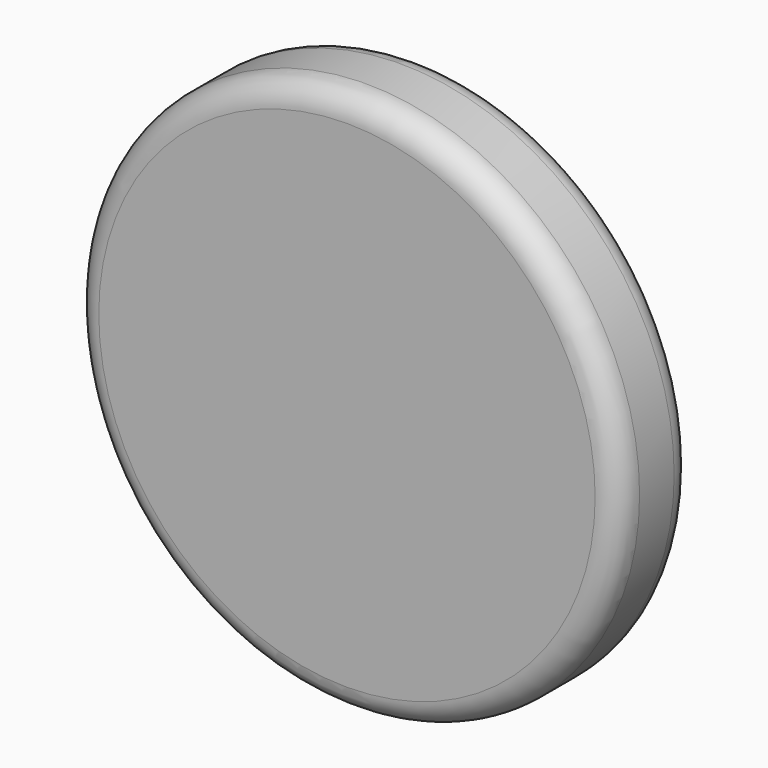
from build123d import *

# Parameters (mm, degrees)
F0_R         = 56.1499717353
F1_DEPTH     = 19.05
F2_R         = 5.08
F3_R         = 5.08
F4_TEXT_SIZE = 7.3197828088
F6_DEPTH     = 12.7
F7_TEXT_SIZE = 6.3348212279
F8_DEPTH     = 12.7


# Not quite as in the source:
# - Text() gives the source's letters only with a copy of the font that has no kerning and outlines rounded to 1/6400 em; it was checked with that copy


with BuildPart() as f1:
    # F0 (on Front) → F1 (new body)
    with BuildSketch(Plane.XZ):
        Circle(F0_R)
    extrude(amount=F1_DEPTH)

    # F2
    f2_edges = [f1.edges().sort_by_distance(p)[0] for p in [
        (-56.149972, -19.05, 0),
    ]]
    fillet(f2_edges, radius=F2_R)

    # F3
    f3_edges = [f1.edges().sort_by_distance(p)[0] for p in [
        (-56.149972, 0, 0),
    ]]
    fillet(f3_edges, radius=F3_R)

    # F4 (on face) → F6 (cut)
    with BuildSketch(Plane(origin=(0, 0, 0), x_dir=(-1, 0, 0), z_dir=(0, 1, 0))):
        with Locations((-15.156253241, 11.1113646999)):
            Text('Palm Tree', F4_TEXT_SIZE, font='Open Sans', text_align=(TextAlign.LEFT, TextAlign.BOTTOM))
    extrude(amount=-F6_DEPTH, mode=Mode.SUBTRACT)

    # F7 (on face) → F8 (cut)
    with BuildSketch(Plane(origin=(0, 0, 0), x_dir=(-1, 0, 0), z_dir=(0, 1, 0))):
        with Locations((-12.0846424252, -4.5610712841)):
            Text('phone Cases', F7_TEXT_SIZE, font='Open Sans', text_align=(TextAlign.LEFT, TextAlign.BOTTOM))
    extrude(amount=-F8_DEPTH, mode=Mode.SUBTRACT)


solid = f1.part
